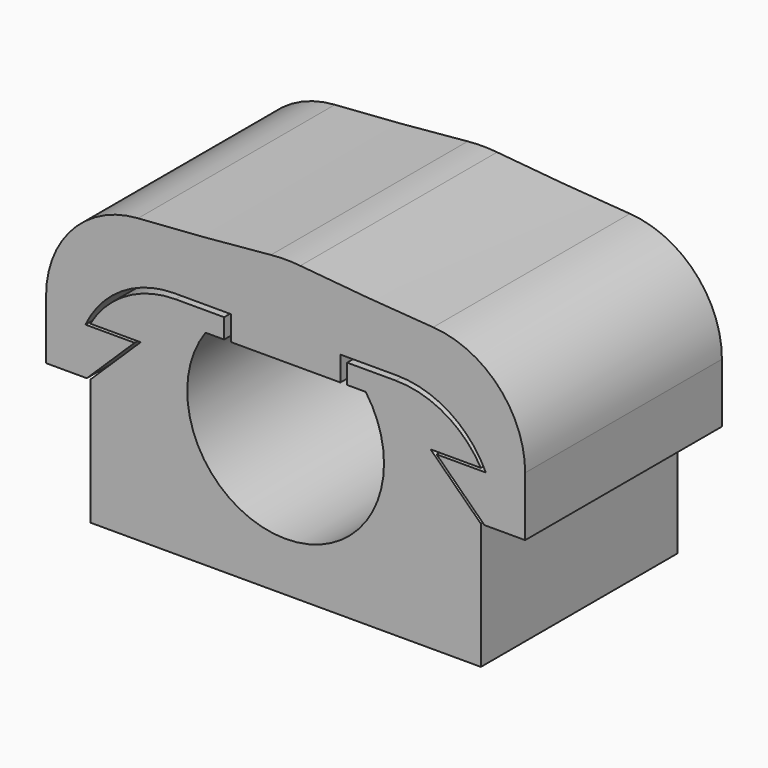
from build123d import *

# Parameters (mm, degrees)
F1_DEPTH      = 5
F2_T1_DEPTH   = 13.6602540378
F2_2_T1_DEPTH = 5
F2_2_T3_DEPTH = 5
F2_2_T5_DEPTH = 15
F2_2_T7_DEPTH = 15
F3_R          = 77.4463937181


# Not quite as in the source:
# - a fillet or chamfer that OpenCascade refuses, or shapes differently, is made with other operations: its cross-section is extruded or revolved along the edge and cut away or added
# - a feature names something its author has since deleted; it is built from what else it names


with BuildPart() as f1:
    # F0 (on Front) → F1 (new body)
    with BuildSketch(Plane.XZ):
        with BuildLine():
            ThreePointArc((1.6283425928, 1.1612494996), (1.9048208821, 0.609637111), (2, 0))
            ThreePointArc((2, 0), (-0.609637111, -1.9048208821), (-1.6283425928, 1.1612494996))
            ThreePointArc((-1.6283425928, 1.1612494996), (-1.4530017276, 1.3743311026), (-1.25, 1.5612494996))
            Line((-1.25, 1.5612494996), (-2.5617376915, 1.5612494996))
            ThreePointArc((-2.5617376915, 1.5612494996), (-2.7993993156, 1.0785932838), (-2.9470322359, 0.5612494996))
            ThreePointArc((-2.9470322359, 0.5612494996), (-2.3112494996, -1.9126227413), (0, -3))
            ThreePointArc((0, -3), (2.1213203436, -2.1213203436), (3, 0))
            ThreePointArc((3, 0), (2.9867287044, 0.2818716839), (2.9470322359, 0.5612494996))
            ThreePointArc((2.9470322359, 0.5612494996), (2.7993993156, 1.0785932838), (2.5617376915, 1.5612494996))
            Line((2.5617376915, 1.5612494996), (1.25, 1.5612494996))
            ThreePointArc((1.25, 1.5612494996), (1.4530017276, 1.3743311026), (1.6283425928, 1.1612494996))
        make_face()
        with BuildLine():
            ThreePointArc((0, -3), (-2.3112494996, -1.9126227413), (-2.9470322359, 0.5612494996))
            Line((-2.9470322359, 0.5612494996), (-3.9696805516, -0.4387505004))
            Line((-3.9696805516, -0.4387505004), (-3.9696805516, -3))
            Line((-3.9696805516, -3), (0, -3))
        make_face()
        with BuildLine():
            ThreePointArc((-2.9470322359, 0.5612494996), (-2.7993993156, 1.0785932838), (-2.5617376915, 1.5612494996))
            Line((-2.5617376915, 1.5612494996), (-3.9696805516, 1.5612494996))
            Line((-3.9696805516, 1.5612494996), (-3.9696805516, 0.5612494996))
            Line((-3.9696805516, 0.5612494996), (-2.9470322359, 0.5612494996))
        make_face()
        with BuildLine():
            Line((3.9696805516, 1.5612494996), (2.5617376915, 1.5612494996))
            ThreePointArc((2.5617376915, 1.5612494996), (2.7993993156, 1.0785932838), (2.9470322359, 0.5612494996))
            Line((2.9470322359, 0.5612494996), (3.9696805516, 0.5612494996))
            Line((3.9696805516, 0.5612494996), (3.9696805516, 1.5612494996))
        make_face()
        with BuildLine():
            Line((3.9696805516, -0.4387505004), (2.9470322359, 0.5612494996))
            ThreePointArc((2.9470322359, 0.5612494996), (2.9867287044, 0.2818716839), (3, 0))
            ThreePointArc((3, 0), (2.1213203436, -2.1213203436), (0, -3))
            Line((0, -3), (3.9696805516, -3))
            Line((3.9696805516, -3), (3.9696805516, -0.4387505004))
        make_face()
        with BuildLine():
            ThreePointArc((-1.25, 1.5612494996), (-1.4530017276, 1.3743311026), (-1.6283425928, 1.1612494996))
            Line((-1.6283425928, 1.1612494996), (-1.25, 1.1612494996))
            Line((-1.25, 1.1612494996), (-1.25, 1.5612494996))
        make_face()
        with BuildLine():
            Line((1.25, 1.1612494996), (1.6283425928, 1.1612494996))
            ThreePointArc((1.6283425928, 1.1612494996), (1.4530017276, 1.3743311026), (1.25, 1.5612494996))
            Line((1.25, 1.5612494996), (1.25, 1.1612494996))
        make_face()
    extrude(amount=F1_DEPTH)

    # F2: fillet of radius 2 on 2 edges, made by hand

    # F2_s2 → F2_t1 (cut)
    with BuildSketch(Plane.XZ.offset(-4.3301270189)):
        with BuildLine():
            ThreePointArc((-2.237629744, 1.5612494996), (-3.237629744, 1.2933003072), (-3.9696805516, 0.5612494996))
            Line((-3.9696805516, 0.5612494996), (-3.9696805516, 1.5612494996))
            Line((-3.9696805516, 1.5612494996), (-2.237629744, 1.5612494996))
        make_face()
        with BuildLine():
            ThreePointArc((3.9696805516, 0.5612494996), (3.237629744, 1.2933003072), (2.237629744, 1.5612494996))
            Line((2.237629744, 1.5612494996), (3.9696805516, 1.5612494996))
            Line((3.9696805516, 1.5612494996), (3.9696805516, 0.5612494996))
        make_face()
    extrude(amount=F2_T1_DEPTH, mode=Mode.SUBTRACT)


with BuildPart() as f1b:
    # F0 (on Front) → F1, piece 2 (new body)
    with BuildSketch(Plane.XZ):
        with BuildLine():
            Line((-4.0696805516, 1.6612494996), (-2.4980492589, 1.6612494996))
            ThreePointArc((-2.4980492589, 1.6612494996), (-1.9105132383, 2.3129935508), (-1.1595288015, 2.7668561507))
            Line((-1.1595288015, 2.7668561507), (-4.8696805516, 2.7668561507))
            Line((-4.8696805516, 2.7668561507), (-4.8696805516, -0.4387505004))
            Line((-4.8696805516, -0.4387505004), (-4.0411964515, -0.4387505004))
            Line((-4.0411964515, -0.4387505004), (-3.9696805516, -0.3688184438))
            Line((-3.9696805516, -0.3688184438), (-3.9696805516, 0.5112494996))
            Line((-3.9696805516, 0.5112494996), (-4.0696805516, 0.5112494996))
            Line((-4.0696805516, 0.5112494996), (-4.0696805516, 1.6612494996))
        make_face()
        Polygon((-3.0696805516, 0.5112494996), (-3.9696805516, 0.5112494996), (-3.9696805516, -0.3688184438), align=None)
        with BuildLine():
            ThreePointArc((-1.1136651652, 1.6612494996), (0, 2), (1.1136651652, 1.6612494996))
            Line((1.1136651652, 1.6612494996), (2.4980492589, 1.6612494996))
            ThreePointArc((2.4980492589, 1.6612494996), (1.9105132383, 2.3129935508), (1.1595288015, 2.7668561507))
            ThreePointArc((1.1595288015, 2.7668561507), (0, 3), (-1.1595288015, 2.7668561507))
            ThreePointArc((-1.1595288015, 2.7668561507), (-1.9105132383, 2.3129935508), (-2.4980492589, 1.6612494996))
            Line((-2.4980492589, 1.6612494996), (-1.1136651652, 1.6612494996))
        make_face()
        with BuildLine():
            ThreePointArc((1.1595288015, 2.7668561507), (1.9105132383, 2.3129935508), (2.4980492589, 1.6612494996))
            Line((2.4980492589, 1.6612494996), (4.0696805516, 1.6612494996))
            Line((4.0696805516, 1.6612494996), (4.0696805516, 0.5112494996))
            Line((4.0696805516, 0.5112494996), (3.9696805516, 0.5112494996))
            Line((3.9696805516, 0.5112494996), (3.9696805516, -0.3688184438))
            Line((3.9696805516, -0.3688184438), (4.0411964515, -0.4387505004))
            Line((4.0411964515, -0.4387505004), (4.8696805516, -0.4387505004))
            Line((4.8696805516, -0.4387505004), (4.8696805516, 2.7668561507))
            Line((4.8696805516, 2.7668561507), (1.1595288015, 2.7668561507))
        make_face()
        Polygon((3.9696805516, -0.3688184438), (3.9696805516, 0.5112494996), (3.0696805516, 0.5112494996), align=None)
        with BuildLine():
            Line((1.1136651652, 1.1612494996), (1.1136651652, 1.6612494996))
            ThreePointArc((1.1136651652, 1.6612494996), (0, 2), (-1.1136651652, 1.6612494996))
            Line((-1.1136651652, 1.6612494996), (-1.1136651652, 1.1612494996))
            Line((-1.1136651652, 1.1612494996), (0, 1.1612494996))
            Line((0, 1.1612494996), (1.1136651652, 1.1612494996))
        make_face()
    extrude(amount=F1_DEPTH)

    # F2#2: fillet of radius 2 on 4 edges, made by hand

    # F2_2_s2 → F2_2_t1 (join)
    with BuildSketch(Plane.XZ):
        with BuildLine():
            ThreePointArc((-4.0696805516, 0.5112494996), (-3.331674382, 1.3494438012), (-2.2592938526, 1.6612494996))
            Line((-2.2592938526, 1.6612494996), (-4.0696805516, 1.6612494996))
            Line((-4.0696805516, 1.6612494996), (-4.0696805516, 0.5112494996))
        make_face()
    extrude(amount=F2_2_T1_DEPTH)

    # F2_2_s4 → F2_2_t3 (join)
    with BuildSketch(Plane.XZ):
        with BuildLine():
            ThreePointArc((2.2592938526, 1.6612494996), (3.331674382, 1.3494438012), (4.0696805516, 0.5112494996))
            Line((4.0696805516, 0.5112494996), (4.0696805516, 1.6612494996))
            Line((4.0696805516, 1.6612494996), (2.2592938526, 1.6612494996))
        make_face()
    extrude(amount=F2_2_T3_DEPTH)

    # F2_2_s6 → F2_2_t5 (cut)
    with BuildSketch(Plane.XZ.offset(-5)):
        with BuildLine():
            ThreePointArc((4.8696805516, 0.7668561507), (4.283894114, 2.181069713), (2.8696805516, 2.7668561507))
            Line((2.8696805516, 2.7668561507), (4.8696805516, 2.7668561507))
            Line((4.8696805516, 2.7668561507), (4.8696805516, 0.7668561507))
        make_face()
    extrude(amount=F2_2_T5_DEPTH, mode=Mode.SUBTRACT)

    # F2_2_s8 → F2_2_t7 (cut)
    with BuildSketch(Plane.XZ.offset(-5)):
        with BuildLine():
            ThreePointArc((-4.8696805516, 0.7668561507), (-4.283894114, 2.181069713), (-2.8696805516, 2.7668561507))
            Line((-2.8696805516, 2.7668561507), (-4.8696805516, 2.7668561507))
            Line((-4.8696805516, 2.7668561507), (-4.8696805516, 0.7668561507))
        make_face()
    extrude(amount=F2_2_T7_DEPTH, mode=Mode.SUBTRACT)

    # F3
    f3_edges = [f1b.edges().sort_by_distance(p)[0] for p in [
        (1.159529, -2.5, 2.766856),
        (-1.159529, -2.5, 2.766856),
    ]]
    fillet(f3_edges, radius=F3_R)


solid = Compound([f1.part, f1b.part])
